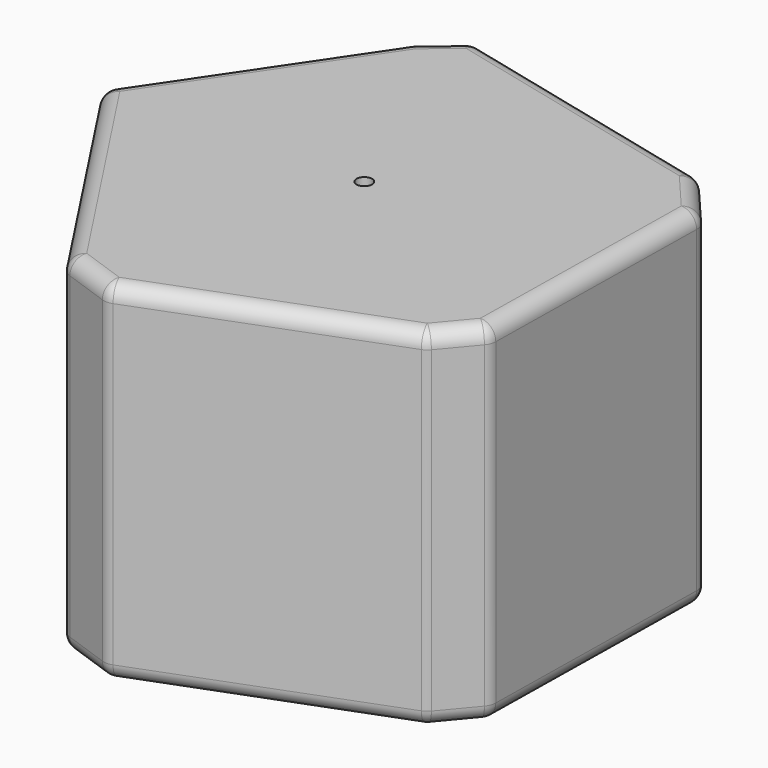
from build123d import *

# Parameters (mm, degrees)
F1_DEPTH      = 45
F3_DEPTH      = 40
F3_TAPER      = 8
F4_R          = 2
F5_T1_DEPTH   = 41
F5_T3_DEPTH   = 35.1069251356
F5_T5_DEPTH   = 6.5937371539
F5_T7_DEPTH   = 31.737863034
F5_T9_DEPTH   = 5.4498579355
F5_T11_DEPTH  = 32.6011890019
F5_T13_DEPTH  = 6.1677770557
F5_T15_DEPTH  = 35.4445627494
F5_T17_DEPTH  = 31.1568553356
F5_T19_DEPTH  = 5.1143087809
F5_T24_DEPTH  = 2
F5_T30_DEPTH  = 2
F5_T36_DEPTH  = 2
F5_T42_DEPTH  = 2
F5_T48_DEPTH  = 2
F5_T54_DEPTH  = 2
F5_T60_DEPTH  = 2
F5_T66_DEPTH  = 2
F5_T72_DEPTH  = 2
F5_T78_DEPTH  = 2
F5_T84_DEPTH  = 2
F5_T90_DEPTH  = 2
F5_T96_DEPTH  = 2
F5_T102_DEPTH = 2
F5_T108_DEPTH = 2
F5_T114_DEPTH = 2
F5_T120_DEPTH = 2
F5_T126_DEPTH = 2
F6_R          = 1
F7_DEPTH      = 45.0010001


# Not quite as in the source:
# - a fillet or chamfer that OpenCascade refuses, or shapes differently, is made with other operations: its cross-section is extruded or revolved along the edge and cut away or added


with BuildPart() as f1:
    # F0 (on Top) → F1 (new body)
    with BuildSketch(Plane.XY):
        Polygon((29.7201480716, -16.6846308857), (30.2449911833, 16.5100768209), (25.0633712858, 22.6006042212), (-10.6668910012, 31.2771238387), (-15.5701944605, 27.1541606635), (-33.9107997715, 0), (-13.3636286482, -31.3134789467), (-6.2161423266, -33.8213965297), (25.438066572, -21.8132548034), align=None)
    extrude(amount=F1_DEPTH)

    # F2 (on Top) → F3 (cut)
    with BuildSketch(Plane.XY):
        Polygon((25, -18.1635632001), (25, 18.1635632001), (-9.5491502813, 29.3892626146), (-30.9016994375, 0), (-9.5491502813, -29.3892626146), align=None)
    extrude(amount=F3_DEPTH, taper=F3_TAPER, mode=Mode.SUBTRACT)

    # F4
    f4_edges = [f1.edges().sort_by_distance(p)[0] for p in [
        (5.988245, 18.429922, 40),
        (22.189183, 16.121385, 20),
        (19.378367, 0, 40),
        (5.988245, -18.429922, 40),
        (-15.677428, -11.390318, 40),
        (-15.677428, 11.390318, 40),
        (-8.475514, 26.084949, 20.000003),
        (-27.427338, 0, 20.000003),
        (-8.475514, -26.084949, 20),
        (22.189183, -16.121385, 20.000003),
    ]]
    fillet(f4_edges, radius=F4_R)

    # F5: fillet of radius 2 on 27 edges, made by hand

    # F5_s2 → F5_t1 (cut)
    with BuildSketch(Plane.XY.offset(2)):
        with BuildLine():
            ThreePointArc((25.4839689775, 22.1062295244), (25.0095176152, 22.5131674422), (24.4326191036, 22.7537722455))
            Line((24.4326191036, 22.7537722455), (25.0633712858, 22.6006042212))
            Line((25.0633712858, 22.6006042212), (25.4839689775, 22.1062295244))
        make_face()
        with BuildLine():
            ThreePointArc((-9.6828471205, 31.0381646067), (-10.6116670526, 31.0417656744), (-11.4419497811, 30.6254124292))
            Line((-11.4419497811, 30.6254124292), (-10.6668910012, 31.2771238387))
            Line((-10.6668910012, 31.2771238387), (-9.6828471205, 31.0381646067))
        make_face()
        with BuildLine():
            ThreePointArc((30.2330765046, 15.75651015), (30.115771586, 16.4637023449), (29.7566283548, 17.0841033313))
            Line((29.7566283548, 17.0841033313), (30.2449911833, 16.5100768209))
            Line((30.2449911833, 16.5100768209), (30.2330765046, 15.75651015))
        make_face()
        with BuildLine():
            ThreePointArc((29.266810806, -17.2275902721), (29.606353406, -16.6423498995), (29.7313303454, -15.9773865656))
            Line((29.7313303454, -15.9773865656), (29.7201480716, -16.6846308857))
            Line((29.7201480716, -16.6846308857), (29.266810806, -17.2275902721))
        make_face()
        with BuildLine():
            ThreePointArc((25.7739373145, -21.4109843833), (25.3988996269, -21.7582581704), (24.9480861633, -21.9991306915))
            Line((24.9480861633, -21.9991306915), (25.438066572, -21.8132548034))
            Line((25.438066572, -21.8132548034), (25.7739373145, -21.4109843833))
        make_face()
        with BuildLine():
            ThreePointArc((-5.5335065177, -33.5624360999), (-6.217763907, -33.6923101567), (-6.90506781, -33.5796656252))
            Line((-6.90506781, -33.5796656252), (-6.2161423266, -33.8213965297))
            Line((-6.2161423266, -33.8213965297), (-5.5335065177, -33.5624360999))
        make_face()
        with BuildLine():
            ThreePointArc((-12.7249750969, -31.5375703823), (-13.294983208, -31.2257163798), (-13.7349453155, -30.7475997522))
            Line((-13.7349453155, -30.7475997522), (-13.3636286482, -31.3134789467))
            Line((-13.3636286482, -31.3134789467), (-12.7249750969, -31.5375703823))
        make_face()
        with BuildLine():
            ThreePointArc((-33.1803118935, -1.1132489554), (-33.5081152827, -0.0026852842), (-33.1655302123, 1.1034079304))
            Line((-33.1655302123, 1.1034079304), (-33.9107997715, 0))
            Line((-33.9107997715, 0), (-33.1803118935, -1.1132489554))
        make_face()
        with BuildLine():
            ThreePointArc((-15.7265735436, 26.922633804), (-15.5557596342, 27.1411687), (-15.3563537075, 27.3339695529))
            Line((-15.3563537075, 27.3339695529), (-15.5701944605, 27.1541606635))
            Line((-15.5701944605, 27.1541606635), (-15.7265735436, 26.922633804))
        make_face()
    extrude(amount=F5_T1_DEPTH, mode=Mode.SUBTRACT)

    # F5_s4 → F5_t3 (cut)
    with BuildSketch(Plane(origin=(17.8543882754, -4.335651076, 0), x_dir=(0, 0, 1), z_dir=(-0.9717588793, 0.235976017, 0))):
        with BuildLine():
            ThreePointArc((0, 25.8766923562), (0.5857864376, 27.2909059185), (2, 27.8766923562))
            Line((2, 27.8766923562), (0, 27.8766923562))
            Line((0, 27.8766923562), (0, 25.8766923562))
        make_face()
        with BuildLine():
            ThreePointArc((43, 27.8766923562), (44.4142135624, 27.2909059185), (45, 25.8766923562))
            Line((45, 25.8766923562), (45, 27.8766923562))
            Line((45, 27.8766923562), (43, 27.8766923562))
        make_face()
    extrude(amount=F5_T3_DEPTH, mode=Mode.SUBTRACT)

    # F5_s6 → F5_t5 (cut)
    with BuildSketch(Plane(origin=(4.0627522572, -4.775399283, 0), x_dir=(0, 0, 1), z_dir=(-0.6479875187, 0.7616509539, 0))):
        with BuildLine():
            ThreePointArc((0, 31.7344500987), (0.5857864376, 33.1486636611), (2, 33.7344500987))
            Line((2, 33.7344500987), (0, 33.7344500987))
            Line((0, 33.7344500987), (0, 31.7344500987))
        make_face()
        with BuildLine():
            ThreePointArc((43, 33.7344500987), (44.4142135624, 33.1486636611), (45, 31.7344500987))
            Line((45, 31.7344500987), (45, 33.7344500987))
            Line((45, 33.7344500987), (43, 33.7344500987))
        make_face()
    extrude(amount=F5_T5_DEPTH, mode=Mode.SUBTRACT)

    # F5_s8 → F5_t7 (cut)
    with BuildSketch(Plane(origin=(-0.2451254322, -15.5034273892, 0), x_dir=(0, 0, 1), z_dir=(0.0158090719, 0.9998750288, 0))):
        with BuildLine():
            ThreePointArc((0, 27.9802024391), (0.5857864376, 29.3944160014), (2, 29.9802024391))
            Line((2, 29.9802024391), (0, 29.9802024391))
            Line((0, 29.9802024391), (0, 27.9802024391))
        make_face()
        with BuildLine():
            ThreePointArc((43, 29.9802024391), (44.4142135624, 29.3944160014), (45, 27.9802024391))
            Line((45, 27.9802024391), (45, 29.9802024391))
            Line((45, 29.9802024391), (43, 29.9802024391))
        make_face()
    extrude(amount=F5_T7_DEPTH, mode=Mode.SUBTRACT)

    # F5_s10 → F5_t9 (cut)
    with BuildSketch(Plane(origin=(0.0534517688, 0.0640188702, 0), x_dir=(0, 0, 1), z_dir=(0.6409109252, 0.7676152591, 0))):
        with BuildLine():
            ThreePointArc((0, 31.5070013796), (0.5857864376, 32.9212149419), (2, 33.5070013796))
            Line((2, 33.5070013796), (0, 33.5070013796))
            Line((0, 33.5070013796), (0, 31.5070013796))
        make_face()
        with BuildLine():
            ThreePointArc((43, 33.5070013796), (44.4142135624, 32.9212149419), (45, 31.5070013796))
            Line((45, 31.5070013796), (45, 33.5070013796))
            Line((45, 33.5070013796), (43, 33.5070013796))
        make_face()
    extrude(amount=F5_T9_DEPTH, mode=Mode.SUBTRACT)

    # F5_s12 → F5_t11 (cut)
    with BuildSketch(Plane(origin=(-15.9676490674, -6.0573869861, 0), x_dir=(0, 0, 1), z_dir=(0.9349840792, 0.3546896835, 0))):
        with BuildLine():
            ThreePointArc((0, 27.4176657385), (0.5857864376, 28.8318793009), (2, 29.4176657385))
            Line((2, 29.4176657385), (0, 29.4176657385))
            Line((0, 29.4176657385), (0, 27.4176657385))
        make_face()
        with BuildLine():
            ThreePointArc((43, 29.4176657385), (44.4142135624, 28.8318793009), (45, 27.4176657385))
            Line((45, 27.4176657385), (45, 29.4176657385))
            Line((45, 29.4176657385), (43, 29.4176657385))
        make_face()
    extrude(amount=F5_T11_DEPTH, mode=Mode.SUBTRACT)

    # F5_s14 → F5_t13 (cut)
    with BuildSketch(Plane(origin=(-1.477173062, 0.5183120511, 0), x_dir=(0, 0, 1), z_dir=(0.9435988419, -0.3310909627, 0))):
        with BuildLine():
            ThreePointArc((0, 31.9719391439), (0.5857864376, 33.3861527063), (2, 33.9719391439))
            Line((2, 33.9719391439), (0, 33.9719391439))
            Line((0, 33.9719391439), (0, 31.9719391439))
        make_face()
        with BuildLine():
            ThreePointArc((43, 33.9719391439), (44.4142135624, 33.3861527063), (45, 31.9719391439))
            Line((45, 31.9719391439), (45, 33.9719391439))
            Line((45, 33.9719391439), (43, 33.9719391439))
        make_face()
    extrude(amount=F5_T13_DEPTH, mode=Mode.SUBTRACT)

    # F5_s16 → F5_t15 (cut)
    with BuildSketch(Plane(origin=(-9.4758761855, 14.4410462956, 0), x_dir=(0, 0, 1), z_dir=(0.5486135269, -0.836076072, 0))):
        with BuildLine():
            ThreePointArc((0, 26.3520082709), (0.5857864376, 27.7662218332), (2, 28.3520082709))
            Line((2, 28.3520082709), (0, 28.3520082709))
            Line((0, 28.3520082709), (0, 26.3520082709))
        make_face()
        with BuildLine():
            ThreePointArc((43, 28.3520082709), (44.4142135624, 27.7662218332), (45, 26.3520082709))
            Line((45, 26.3520082709), (45, 28.3520082709))
            Line((45, 28.3520082709), (43, 28.3520082709))
        make_face()
    extrude(amount=F5_T15_DEPTH, mode=Mode.SUBTRACT)

    # F5_s18 → F5_t17 (cut)
    with BuildSketch(Plane(origin=(7.5606241791, 11.1938728407, 0), x_dir=(0, 0, 1), z_dir=(-0.5597149161, -0.8286852314, 0))):
        with BuildLine():
            ThreePointArc((0, 26.1013789558), (0.5857864376, 27.5155925181), (2, 28.1013789558))
            Line((2, 28.1013789558), (0, 28.1013789558))
            Line((0, 28.1013789558), (0, 26.1013789558))
        make_face()
        with BuildLine():
            ThreePointArc((43, 28.1013789558), (44.4142135624, 27.5155925181), (45, 26.1013789558))
            Line((45, 26.1013789558), (45, 28.1013789558))
            Line((45, 28.1013789558), (43, 28.1013789558))
        make_face()
    extrude(amount=F5_T17_DEPTH, mode=Mode.SUBTRACT)

    # F5_s20 → F5_t19 (cut)
    with BuildSketch(Plane(origin=(8.3826927124, 7.0486221481, 0), x_dir=(0, 0, 1), z_dir=(-0.7653827905, -0.6435753134, 0))):
        with BuildLine():
            ThreePointArc((0, 28.803920042), (0.5857864376, 30.2181336044), (2, 30.803920042))
            Line((2, 30.803920042), (0, 30.803920042))
            Line((0, 30.803920042), (0, 28.803920042))
        make_face()
        with BuildLine():
            ThreePointArc((43, 30.803920042), (44.4142135624, 30.2181336044), (45, 28.803920042))
            Line((45, 28.803920042), (45, 30.803920042))
            Line((45, 30.803920042), (43, 30.803920042))
        make_face()
    extrude(amount=F5_T19_DEPTH, mode=Mode.SUBTRACT)


with BuildPart() as f5_tool22:
    # F5_s23 → F5_t24 (new body)
    with BuildSketch(Plane.XY.offset(2)):
        Polygon((23.9606670696, 20.810254487), (24.4326191036, 22.7537722455), (25.0633712858, 22.6006042212), (25.4839689775, 22.1062295244), align=None)
    extrude(amount=-F5_T24_DEPTH)

    # F5_s25 → F5_t26 (revolve, cut)
    with BuildSketch(Plane(origin=(23.9606670696, 20.810254487, 2), x_dir=(-0.5244252728, -0.8514564776, 0), z_dir=(0.8514564776, -0.5244252728, 0))):
        with BuildLine():
            ThreePointArc((0, -2), (2, 0), (0, 2))
            Line((0, 2), (0, -2))
        make_face()
    revolve(axis=Axis((23.9606670696, 20.810254487, 2), (0, 0, -1)), mode=Mode.SUBTRACT)


with BuildPart() as f1_1:
    add(f1.part)

    # F5_t21: cut F5_tool22
    add(f5_tool22.part, mode=Mode.SUBTRACT)


with BuildPart() as f5_tool28:
    # F5_s29 → F5_t30 (new body)
    with BuildSketch(Plane.XY.offset(43)):
        Polygon((23.9606670696, 20.810254487), (25.4839689775, 22.1062295244), (25.0633712858, 22.6006042212), (24.4326191036, 22.7537722455), align=None)
    extrude(amount=F5_T30_DEPTH)

    # F5_s31 → F5_t32 (revolve, cut)
    with BuildSketch(Plane(origin=(23.9606670696, 20.810254487, 43), x_dir=(-0.5244252728, -0.8514564776, 0), z_dir=(-0.8514564776, 0.5244252728, 0))):
        with BuildLine():
            ThreePointArc((0, -2), (2, 0), (0, 2))
            Line((0, 2), (0, -2))
        make_face()
    revolve(axis=Axis((23.9606670696, 20.810254487, 43), (0, 0, 1)), mode=Mode.SUBTRACT)


with BuildPart() as f1_2:
    add(f1_1.part)

    # F5_t27: cut F5_tool28
    add(f5_tool28.part, mode=Mode.SUBTRACT)


with BuildPart() as f5_tool34:
    # F5_s35 → F5_t36 (new body)
    with BuildSketch(Plane.XY.offset(2)):
        Polygon((-10.1547991544, 29.0946468482), (-9.6828471205, 31.0381646067), (-10.6668910012, 31.2771238387), (-11.4419497811, 30.6254124292), align=None)
    extrude(amount=-F5_T36_DEPTH)

    # F5_s37 → F5_t38 (revolve, cut)
    with BuildSketch(Plane(origin=(-10.1547991544, 29.0946468482, 2), x_dir=(0.2284339491, -0.9735594131, 0), z_dir=(0.9735594131, 0.2284339491, 0))):
        with BuildLine():
            ThreePointArc((0, -2), (2, 0), (0, 2))
            Line((0, 2), (0, -2))
        make_face()
    revolve(axis=Axis((-10.1547991544, 29.0946468482, 2), (0, 0, -1)), mode=Mode.SUBTRACT)


with BuildPart() as f1_3:
    add(f1_2.part)

    # F5_t33: cut F5_tool34
    add(f5_tool34.part, mode=Mode.SUBTRACT)


with BuildPart() as f5_tool40:
    # F5_s41 → F5_t42 (new body)
    with BuildSketch(Plane.XY.offset(43)):
        Polygon((-10.1547991544, 29.0946468482), (-9.6828471205, 31.0381646067), (-10.6668910012, 31.2771238387), (-11.4419497811, 30.6254124292), align=None)
    extrude(amount=F5_T42_DEPTH)

    # F5_s43 → F5_t44 (revolve, cut)
    with BuildSketch(Plane(origin=(-10.1547991544, 29.0946468482, 43), x_dir=(0.2284339491, -0.9735594131, 0), z_dir=(-0.9735594131, -0.2284339491, 0))):
        with BuildLine():
            ThreePointArc((0, -2), (2, 0), (0, 2))
            Line((0, 2), (0, -2))
        make_face()
    revolve(axis=Axis((-10.1547991544, 29.0946468482, 43), (0, 0, 1)), mode=Mode.SUBTRACT)


with BuildPart() as f1_4:
    add(f1_3.part)

    # F5_t39: cut F5_tool40
    add(f5_tool40.part, mode=Mode.SUBTRACT)


with BuildPart() as f5_tool46:
    # F5_s47 → F5_t48 (new body)
    with BuildSketch(Plane.XY.offset(2)):
        Polygon((28.233326447, 15.7881282939), (30.2330765046, 15.75651015), (30.2449911833, 16.5100768209), (29.7566283548, 17.0841033313), align=None)
    extrude(amount=-F5_T48_DEPTH)

    # F5_s49 → F5_t50 (revolve, cut)
    with BuildSketch(Plane(origin=(28.233326447, 15.7881282939, 2), x_dir=(-0.9412225695, -0.3377870255, 0), z_dir=(0.3377870255, -0.9412225695, 0))):
        with BuildLine():
            ThreePointArc((0, -2), (2, 0), (0, 2))
            Line((0, 2), (0, -2))
        make_face()
    revolve(axis=Axis((28.233326447, 15.7881282939, 2), (0, 0, -1)), mode=Mode.SUBTRACT)


with BuildPart() as f1_5:
    add(f1_4.part)

    # F5_t45: cut F5_tool46
    add(f5_tool46.part, mode=Mode.SUBTRACT)


with BuildPart() as f5_tool52:
    # F5_s53 → F5_t54 (new body)
    with BuildSketch(Plane.XY.offset(43)):
        Polygon((28.233326447, 15.7881282939), (29.7566283548, 17.0841033313), (30.2449911833, 16.5100768209), (30.2330765046, 15.75651015), align=None)
    extrude(amount=F5_T54_DEPTH)

    # F5_s55 → F5_t56 (revolve, cut)
    with BuildSketch(Plane(origin=(28.233326447, 15.7881282939, 43), x_dir=(-0.9412225695, -0.3377870255, 0), z_dir=(-0.3377870255, 0.9412225695, 0))):
        with BuildLine():
            ThreePointArc((0, -2), (2, 0), (0, 2))
            Line((0, 2), (0, -2))
        make_face()
    revolve(axis=Axis((28.233326447, 15.7881282939, 43), (0, 0, 1)), mode=Mode.SUBTRACT)


with BuildPart() as f1_6:
    add(f1_5.part)

    # F5_t51: cut F5_tool52
    add(f5_tool52.part, mode=Mode.SUBTRACT)


with BuildPart() as f5_tool58:
    # F5_s59 → F5_t60 (new body)
    with BuildSketch(Plane.XY.offset(2)):
        Polygon((27.7315802878, -15.9457684217), (29.266810806, -17.2275902721), (29.7201480716, -16.6846308857), (29.7313303454, -15.9773865656), align=None)
    extrude(amount=-F5_T60_DEPTH)

    # F5_s61 → F5_t62 (revolve, cut)
    with BuildSketch(Plane(origin=(27.7315802878, -15.9457684217, 2), x_dir=(-0.9373865591, 0.3482907389, 0), z_dir=(-0.3482907389, -0.9373865591, 0))):
        with BuildLine():
            ThreePointArc((0, -2), (2, 0), (0, 2))
            Line((0, 2), (0, -2))
        make_face()
    revolve(axis=Axis((27.7315802878, -15.9457684217, 2), (0, 0, -1)), mode=Mode.SUBTRACT)


with BuildPart() as f1_7:
    add(f1_6.part)

    # F5_t57: cut F5_tool58
    add(f5_tool58.part, mode=Mode.SUBTRACT)


with BuildPart() as f5_tool64:
    # F5_s65 → F5_t66 (new body)
    with BuildSketch(Plane.XY.offset(43)):
        Polygon((27.7315802878, -15.9457684217), (29.266810806, -17.2275902721), (29.7201480716, -16.6846308857), (29.7313303454, -15.9773865656), align=None)
    extrude(amount=F5_T66_DEPTH)

    # F5_s67 → F5_t68 (revolve, cut)
    with BuildSketch(Plane(origin=(27.7315802878, -15.9457684217, 43), x_dir=(-0.9373865591, 0.3482907389, 0), z_dir=(0.3482907389, 0.9373865591, 0))):
        with BuildLine():
            ThreePointArc((0, -2), (2, 0), (0, 2))
            Line((0, 2), (0, -2))
        make_face()
    revolve(axis=Axis((27.7315802878, -15.9457684217, 43), (0, 0, 1)), mode=Mode.SUBTRACT)


with BuildPart() as f1_8:
    add(f1_7.part)

    # F5_t63: cut F5_tool64
    add(f5_tool64.part, mode=Mode.SUBTRACT)


with BuildPart() as f5_tool70:
    # F5_s71 → F5_t72 (new body)
    with BuildSketch(Plane.XY.offset(2)):
        Polygon((24.2387067963, -20.129162533), (25.7739373145, -21.4109843833), (25.438066572, -21.8132548034), (24.9480861633, -21.9991306915), align=None)
    extrude(amount=-F5_T72_DEPTH)

    # F5_s73 → F5_t74 (revolve, cut)
    with BuildSketch(Plane(origin=(24.2387067963, -20.129162533, 2), x_dir=(-0.5800964153, 0.8145478187, 0), z_dir=(-0.8145478187, -0.5800964153, 0))):
        with BuildLine():
            ThreePointArc((0, -2), (2, 0), (0, 2))
            Line((0, 2), (0, -2))
        make_face()
    revolve(axis=Axis((24.2387067963, -20.129162533, 2), (0, 0, -1)), mode=Mode.SUBTRACT)


with BuildPart() as f1_9:
    add(f1_8.part)

    # F5_t69: cut F5_tool70
    add(f5_tool70.part, mode=Mode.SUBTRACT)


with BuildPart() as f5_tool76:
    # F5_s77 → F5_t78 (new body)
    with BuildSketch(Plane.XY.offset(43)):
        Polygon((24.2387067963, -20.129162533), (25.7739373145, -21.4109843833), (25.438066572, -21.8132548034), (24.9480861633, -21.9991306915), align=None)
    extrude(amount=F5_T78_DEPTH)

    # F5_s79 → F5_t80 (revolve, cut)
    with BuildSketch(Plane(origin=(24.2387067963, -20.129162533, 43), x_dir=(-0.5800964153, 0.8145478187, 0), z_dir=(0.8145478187, 0.5800964153, 0))):
        with BuildLine():
            ThreePointArc((0, -2), (2, 0), (0, 2))
            Line((0, 2), (0, -2))
        make_face()
    revolve(axis=Axis((24.2387067963, -20.129162533, 43), (0, 0, 1)), mode=Mode.SUBTRACT)


with BuildPart() as f1_10:
    add(f1_9.part)

    # F5_t75: cut F5_tool76
    add(f5_tool76.part, mode=Mode.SUBTRACT)


with BuildPart() as f5_tool82:
    # F5_s83 → F5_t84 (new body)
    with BuildSketch(Plane.XY.offset(2)):
        Polygon((-6.2428858846, -31.6924679414), (-5.5335065177, -33.5624360999), (-6.2161423266, -33.8213965297), (-6.90506781, -33.5796656252), align=None)
    extrude(amount=-F5_T84_DEPTH)

    # F5_s85 → F5_t86 (revolve, cut)
    with BuildSketch(Plane(origin=(-6.2428858846, -31.6924679414, 2), x_dir=(-0.0125609888, 0.9999211077, 0), z_dir=(-0.9999211077, -0.0125609888, 0))):
        with BuildLine():
            ThreePointArc((0, -2), (2, 0), (0, 2))
            Line((0, 2), (0, -2))
        make_face()
    revolve(axis=Axis((-6.2428858846, -31.6924679414, 2), (0, 0, -1)), mode=Mode.SUBTRACT)


with BuildPart() as f1_11:
    add(f1_10.part)

    # F5_t81: cut F5_tool82
    add(f5_tool82.part, mode=Mode.SUBTRACT)


with BuildPart() as f5_tool88:
    # F5_s89 → F5_t90 (new body)
    with BuildSketch(Plane.XY.offset(43)):
        Polygon((-6.2428858846, -31.6924679414), (-5.5335065177, -33.5624360999), (-6.2161423266, -33.8213965297), (-6.90506781, -33.5796656252), align=None)
    extrude(amount=F5_T90_DEPTH)

    # F5_s91 → F5_t92 (revolve, cut)
    with BuildSketch(Plane(origin=(-6.2428858846, -31.6924679414, 43), x_dir=(-0.0125609888, 0.9999211077, 0), z_dir=(0.9999211077, 0.0125609888, 0))):
        with BuildLine():
            ThreePointArc((0, -2), (2, 0), (0, 2))
            Line((0, 2), (0, -2))
        make_face()
    revolve(axis=Axis((-6.2428858846, -31.6924679414, 43), (0, 0, 1)), mode=Mode.SUBTRACT)


with BuildPart() as f1_12:
    add(f1_11.part)

    # F5_t87: cut F5_tool88
    add(f5_tool88.part, mode=Mode.SUBTRACT)


with BuildPart() as f5_tool94:
    # F5_s95 → F5_t96 (new body)
    with BuildSketch(Plane.XY.offset(2)):
        Polygon((-12.0627931715, -29.6503726985), (-12.7249750969, -31.5375703823), (-13.3636286482, -31.3134789467), (-13.7349453155, -30.7475997522), align=None)
    extrude(amount=-F5_T96_DEPTH)

    # F5_s97 → F5_t98 (revolve, cut)
    with BuildSketch(Plane(origin=(-12.0627931715, -29.6503726985, 2), x_dir=(0.6160950182, 0.7876718406, 0), z_dir=(-0.7876718406, 0.6160950182, 0))):
        with BuildLine():
            ThreePointArc((0, -2), (2, 0), (0, 2))
            Line((0, 2), (0, -2))
        make_face()
    revolve(axis=Axis((-12.0627931715, -29.6503726985, 2), (0, 0, -1)), mode=Mode.SUBTRACT)


with BuildPart() as f1_13:
    add(f1_12.part)

    # F5_t93: cut F5_tool94
    add(f5_tool94.part, mode=Mode.SUBTRACT)


with BuildPart() as f5_tool100:
    # F5_s101 → F5_t102 (new body)
    with BuildSketch(Plane.XY.offset(43)):
        Polygon((-12.0627931715, -29.6503726985), (-13.7349453155, -30.7475997522), (-13.3636286482, -31.3134789467), (-12.7249750969, -31.5375703823), align=None)
    extrude(amount=F5_T102_DEPTH)

    # F5_s103 → F5_t104 (revolve, cut)
    with BuildSketch(Plane(origin=(-12.0627931715, -29.6503726985, 43), x_dir=(0.6160950182, 0.7876718406, 0), z_dir=(0.7876718406, -0.6160950182, 0))):
        with BuildLine():
            ThreePointArc((0, -2), (2, 0), (0, 2))
            Line((0, 2), (0, -2))
        make_face()
    revolve(axis=Axis((-12.0627931715, -29.6503726985, 43), (0, 0, 1)), mode=Mode.SUBTRACT)


with BuildPart() as f1_14:
    add(f1_13.part)

    # F5_t99: cut F5_tool100
    add(f5_tool100.part, mode=Mode.SUBTRACT)


with BuildPart() as f5_tool106:
    # F5_s107 → F5_t108 (new body)
    with BuildSketch(Plane.XY.offset(2)):
        Polygon((-31.5081597495, -0.0160219017), (-33.1655302123, 1.1034079304), (-33.9107997715, 0), (-33.1803118935, -1.1132489554), align=None)
    extrude(amount=-F5_T108_DEPTH)

    # F5_s109 → F5_t110 (revolve, cut)
    with BuildSketch(Plane(origin=(-31.5081597495, -0.0160219017, 2), x_dir=(0.9999777666, -0.0066683088, 0), z_dir=(0.0066683088, 0.9999777666, 0))):
        with BuildLine():
            ThreePointArc((0, -2), (2, 0), (0, 2))
            Line((0, 2), (0, -2))
        make_face()
    revolve(axis=Axis((-31.5081597495, -0.0160219017, 2), (0, 0, -1)), mode=Mode.SUBTRACT)


with BuildPart() as f1_15:
    add(f1_14.part)

    # F5_t105: cut F5_tool106
    add(f5_tool106.part, mode=Mode.SUBTRACT)


with BuildPart() as f5_tool112:
    # F5_s113 → F5_t114 (new body)
    with BuildSketch(Plane.XY.offset(43)):
        Polygon((-31.5081597495, -0.0160219017), (-33.1803118935, -1.1132489554), (-33.9107997715, 0), (-33.1655302123, 1.1034079304), align=None)
    extrude(amount=F5_T114_DEPTH)

    # F5_s115 → F5_t116 (revolve, cut)
    with BuildSketch(Plane(origin=(-31.5081597495, -0.0160219017, 43), x_dir=(0.9999777666, -0.0066683088, 0), z_dir=(-0.0066683088, -0.9999777666, 0))):
        with BuildLine():
            ThreePointArc((0, -2), (2, 0), (0, 2))
            Line((0, 2), (0, -2))
        make_face()
    revolve(axis=Axis((-31.5081597495, -0.0160219017, 43), (0, 0, 1)), mode=Mode.SUBTRACT)


with BuildPart() as f1_16:
    add(f1_15.part)

    # F5_t111: cut F5_tool112
    add(f5_tool112.part, mode=Mode.SUBTRACT)


with BuildPart() as f5_tool118:
    # F5_s119 → F5_t120 (new body)
    with BuildSketch(Plane.XY.offset(2)):
        Polygon((-14.0692030808, 25.8032039719), (-15.7265735436, 26.922633804), (-15.5701944605, 27.1541606635), (-15.3563537075, 27.3339695529), align=None)
    extrude(amount=-F5_T120_DEPTH)

    # F5_s121 → F5_t122 (revolve, cut)
    with BuildSketch(Plane(origin=(-14.0692030808, 25.8032039719, 2), x_dir=(0.7432782767, -0.6689823641, 0), z_dir=(0.6689823641, 0.7432782767, 0))):
        with BuildLine():
            ThreePointArc((0, -2), (2, 0), (0, 2))
            Line((0, 2), (0, -2))
        make_face()
    revolve(axis=Axis((-14.0692030808, 25.8032039719, 2), (0, 0, -1)), mode=Mode.SUBTRACT)


with BuildPart() as f1_17:
    add(f1_16.part)

    # F5_t117: cut F5_tool118
    add(f5_tool118.part, mode=Mode.SUBTRACT)


with BuildPart() as f5_tool124:
    # F5_s125 → F5_t126 (new body)
    with BuildSketch(Plane.XY.offset(43)):
        Polygon((-14.0692030808, 25.8032039719), (-15.7265735436, 26.922633804), (-15.5701944605, 27.1541606635), (-15.3563537075, 27.3339695529), align=None)
    extrude(amount=F5_T126_DEPTH)

    # F5_s127 → F5_t128 (revolve, cut)
    with BuildSketch(Plane(origin=(-14.0692030808, 25.8032039719, 43), x_dir=(0.7432782767, -0.6689823641, 0), z_dir=(-0.6689823641, -0.7432782767, 0))):
        with BuildLine():
            ThreePointArc((0, -2), (2, 0), (0, 2))
            Line((0, 2), (0, -2))
        make_face()
    revolve(axis=Axis((-14.0692030808, 25.8032039719, 43), (0, 0, 1)), mode=Mode.SUBTRACT)


with BuildPart() as f1_18:
    add(f1_17.part)

    # F5_t123: cut F5_tool124
    add(f5_tool124.part, mode=Mode.SUBTRACT)

    # F6 (on face) → F7 (cut, through all)
    with BuildSketch(Plane.XY.offset(45)):
        Circle(F6_R)
    extrude(amount=-F7_DEPTH, mode=Mode.SUBTRACT)


solid = f1_18.part
